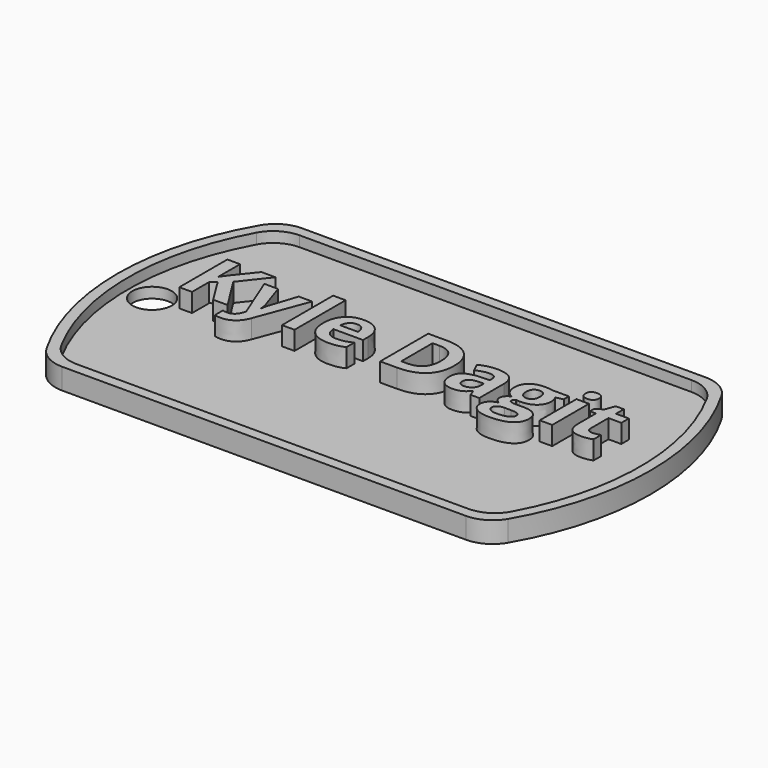
from build123d import *

# Parameters (mm, degrees)
F0_R         = 1.8739594118
F1_DEPTH     = 1
F3_DEPTH     = 1
F4_TEXT_SIZE = 8.0120904992
F5_DEPTH     = 1.778


# Not quite as in the source:
# - Text() gives the source's letters only with a copy of the font that has no kerning and outlines rounded to 1/6400 em; it was checked with that copy


with BuildPart() as f1:
    # F0 (on Top) → F1 (new body)
    with BuildSketch(Plane.XY):
        with BuildLine():
            ThreePointArc((-19.2474145991, 14.2875), (-20.8349145991, 13.862130657), (-21.9970452561, 12.7))
            ThreePointArc((-21.9970452561, 12.7), (-25.4, 0), (-21.9970452561, -12.7))
            ThreePointArc((-21.9970452561, -12.7), (-20.8349145991, -13.862130657), (-19.2474145991, -14.2875))
            Line((-19.2474145991, -14.2875), (19.2474145991, -14.2875))
            ThreePointArc((19.2474145991, -14.2875), (20.8349145991, -13.862130657), (21.9970452561, -12.7))
            ThreePointArc((21.9970452561, -12.7), (25.4, 0), (21.9970452561, 12.7))
            ThreePointArc((21.9970452561, 12.7), (20.8349145991, 13.862130657), (19.2474145991, 14.2875))
            Line((19.2474145991, 14.2875), (-19.2474145991, 14.2875))
        make_face()
        with Locations((-22.0978986472, 0)):
            Circle(F0_R, mode=Mode.SUBTRACT)
    extrude(amount=F1_DEPTH)

    # F2 (on face) → F3 (join)
    with BuildSketch(Plane.XY.offset(1)):
        with BuildLine():
            Line((19.2474145991, 14.2875), (-19.2474145991, 14.2875))
            ThreePointArc((-19.2474145991, 14.2875), (-20.8349145991, 13.862130657), (-21.9970452561, 12.7))
            ThreePointArc((-21.9970452561, 12.7), (-25.4, 0), (-21.9970452561, -12.7))
            ThreePointArc((-21.9970452561, -12.7), (-20.8349145991, -13.862130657), (-19.2474145991, -14.2875))
            Line((-19.2474145991, -14.2875), (19.2474145991, -14.2875))
            ThreePointArc((19.2474145991, -14.2875), (20.8349145991, -13.862130657), (21.9970452561, -12.7))
            ThreePointArc((21.9970452561, -12.7), (25.4, 0), (21.9970452561, 12.7))
            ThreePointArc((21.9970452561, 12.7), (20.8349145991, 13.862130657), (19.2474145991, 14.2875))
        make_face()
        with BuildLine():
            ThreePointArc((-21.4526124879, 11.6252061249), (-20.2856017842, 12.8404540819), (-18.6611352482, 13.2875))
            Line((-18.6611352482, 13.2875), (18.6611352482, 13.2875))
            ThreePointArc((18.6611352482, 13.2875), (20.2856017842, 12.8404540819), (21.4526124879, 11.6252061249))
            ThreePointArc((21.4526124879, 11.6252061249), (24.4, 0), (21.4526124879, -11.6252061249))
            ThreePointArc((21.4526124879, -11.6252061249), (20.2856017842, -12.8404540819), (18.6611352482, -13.2875))
            Line((18.6611352482, -13.2875), (-18.6611352482, -13.2875))
            ThreePointArc((-18.6611352482, -13.2875), (-20.2856017842, -12.8404540819), (-21.4526124879, -11.6252061249))
            ThreePointArc((-21.4526124879, -11.6252061249), (-24.4, 0), (-21.4526124879, 11.6252061249))
        make_face(mode=Mode.SUBTRACT)
    extrude(amount=F3_DEPTH)

    # F4 (on face) → F5 (join)
    with BuildSketch(Plane.XY.offset(1)):
        with Locations((-20.2239392354, 0)):
            Text('Kyle Dagit', F4_TEXT_SIZE, font='Open Sans', font_style=FontStyle.BOLD, text_align=(TextAlign.LEFT, TextAlign.BOTTOM))
    extrude(amount=F5_DEPTH)


solid = f1.part
